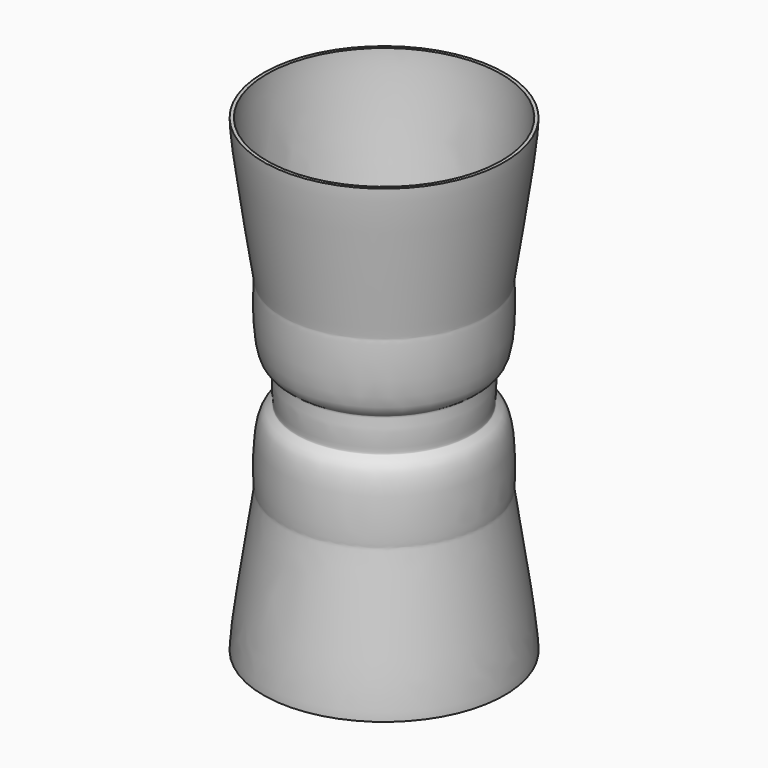
from build123d import *


# Not quite as in the source:
# - the dataset's text gives a spline's control points without its knots; the knots are read off the source's solid


with BuildPart() as f1:
    # F0 (on Front) → F1 (revolve)
    with BuildSketch(Plane.XZ):
        with BuildLine():
            add(Edge.make_bspline(
                [(-25.6999999929, 49.9995985946), (-25.6999852443, 49.5815721843), (-25.6538749277, 48.5653157161), (-25.4124525948, 45.8668468324), (-24.878392708, 41.4753136074), (-24.1648894445, 36.3890603498), (-23.5646349571, 32.3122072602), (-23.1193375058, 29.352931232), (-22.6985490396, 26.594557592), (-22.3219193496, 24.139852673), (-22.0091222222, 22.0915768733), (-21.8182230906, 20.8108258495), (-21.7174489533, 20.0942392935), (-21.67125295, 19.7339820401), (-21.6557990976, 19.5482726937), (-21.6565288364, 19.4907810276), (-21.6608822965, 19.4278153928), (-21.6708680053, 19.3301556268), (-21.6927063082, 19.1336817496), (-21.7207099556, 18.7606404993), (-21.7568005161, 18.0992294459), (-21.7964158924, 16.9880468241), (-21.8179345694, 15.3198351183), (-21.796108146, 13.4398535012), (-21.7132440964, 11.4715337789), (-21.5509831384, 9.5365922757), (-21.3331419094, 8.0502720792), (-21.0956507165, 6.9899388657), (-20.9159406074, 6.3893416768), (-20.7487018006, 5.9506466857), (-20.5613811169, 5.5380982544), (-20.2931757466, 5.0927515424), (-19.9384796595, 4.6682731625), (-19.5759422383, 4.3410734286), (-19.2352502373, 4.0939290526), (-18.9441027544, 3.9056385832), (-18.727928559, 3.7593647128), (-18.6286459873, 3.6717813487), (-18.5923884128, 3.6276224499), (-18.5741459494, 3.5991000841), (-18.5413846399, 3.5234207305), (-18.5092785415, 3.3386711833), (-18.5010370978, 3.0632052381), (-18.5186377506, 2.7098792723), (-18.5683738347, 2.1473494462), (-18.657056361, 1.2888816597), (-18.7, 0.453140888), (-18.7, 0)],
                knots=[1e-05, 1e-05, 1e-05, 1e-05, 0.03125, 0.0625, 0.125, 0.1875, 0.21875, 0.25, 0.28125, 0.3125, 0.34375, 0.375, 0.390625, 0.40625, 0.421875, 0.4375, 0.4453125, 0.453125, 0.46875, 0.484375, 0.5, 0.53125, 0.5625, 0.59375, 0.625, 0.65625, 0.6875, 0.703125, 0.71875, 0.7265625, 0.734375, 0.75, 0.765625, 0.78125, 0.796875, 0.8125, 0.828125, 0.84375, 0.8515625, 0.859375, 0.875, 0.890625, 0.90625, 0.921875, 0.9375, 0.96875, 1, 1, 1, 1], degree=3))
            Line((-18.7, 0), (-18, 0))
            add(Edge.make_bspline(
                [(-25, 50), (-25, 45), (-20.7458853577, 19.1793841739), (-21.079257979, 19.6349945691), (-21.4844424281, 4.9074373991), (-17.1919062111, 4.4391883758), (-18, 2), (-18, 0)],
                knots=[0, 0, 0, 0, 0.3988240253, 0.4713189234, 0.7330888037, 0.8550102037, 1, 1, 1, 1], degree=3))
            Line((-25, 50), (-25.6999999928, 49.9995985946))
        make_face()
        with BuildLine():
            Line((-25.7, -50), (-25, -50))
            add(Edge.make_bspline(
                [(-25, -50), (-25, -45), (-20.7458853577, -19.1793841739), (-21.079257979, -19.6349945691), (-21.3761518713, -8.8435592571), (-20, -6)],
                knots=[0, 0, 0, 0, 0.3988240253, 0.4713189234, 0.7330888037, 0.7330888037, 0.7330888037, 0.7330888037], degree=3))
            add(Edge.make_bspline(
                [(-20, -6), (-19.5032922638, -4.9736467966), (-18.7970130134, -4.6778168777), (-18.3324850568, -4.3324850568)],
                knots=[0.7330888037, 0.7330888037, 0.7330888037, 0.7330888037, 0.8275719254, 0.8275719254, 0.8275719254, 0.8275719254], degree=3))
            Line((-18.3324850568, -4.3324850568), (-18, -4))
            add(Edge.make_bspline(
                [(-18, -4), (-17.5610324502, -3.3250003398), (-18, -2), (-18, 0)],
                knots=[0.8550102037, 0.8550102037, 0.8550102037, 0.8550102037, 1, 1, 1, 1], degree=3))
            Line((-18, 0), (-18.7, 0))
            add(Edge.make_bspline(
                [(-25.7, -50), (-25.7, -49.5818974293), (-25.653894243, -48.5655316105), (-25.4124525948, -45.8668468324), (-24.878392708, -41.4753136074), (-24.1648894445, -36.3890603498), (-23.5646349571, -32.3122072602), (-23.1193375058, -29.352931232), (-22.6985490396, -26.594557592), (-22.3219193496, -24.139852673), (-22.0091222222, -22.0915768733), (-21.8182230906, -20.8108258495), (-21.7174489533, -20.0942392935), (-21.67125295, -19.7339820401), (-21.6557990976, -19.5482726937), (-21.6565288364, -19.4907810276), (-21.6608822965, -19.4278153928), (-21.6708680053, -19.3301556268), (-21.6927063082, -19.1336817496), (-21.7207099556, -18.7606404993), (-21.7568005161, -18.0992294459), (-21.7964158924, -16.9880468241), (-21.8179345694, -15.3198351183), (-21.796108146, -13.4398535012), (-21.7132440964, -11.4715337789), (-21.5509831384, -9.5365922757), (-21.3331419094, -8.0502720792), (-21.0956507165, -6.9899388657), (-20.9159406074, -6.3893416768), (-20.7487018006, -5.9506466857), (-20.5613811169, -5.5380982544), (-20.2931757466, -5.0927515424), (-19.9384796595, -4.6682731625), (-19.5759422383, -4.3410734286), (-19.2352502373, -4.0939290526), (-18.9441027544, -3.9056385832), (-18.727928559, -3.7593647128), (-18.6286459873, -3.6717813487), (-18.5923884128, -3.6276224499), (-18.5741459494, -3.5991000841), (-18.5413846399, -3.5234207305), (-18.5092785415, -3.3386711833), (-18.5010370978, -3.0632052381), (-18.5186377506, -2.7098792723), (-18.5683738347, -2.1473494462), (-18.657056361, -1.2888816597), (-18.7, -0.453140888), (-18.7, 0)],
                knots=[0, 0, 0, 0, 0.03125, 0.0625, 0.125, 0.1875, 0.21875, 0.25, 0.28125, 0.3125, 0.34375, 0.375, 0.390625, 0.40625, 0.421875, 0.4375, 0.4453125, 0.453125, 0.46875, 0.484375, 0.5, 0.53125, 0.5625, 0.59375, 0.625, 0.65625, 0.6875, 0.703125, 0.71875, 0.7265625, 0.734375, 0.75, 0.765625, 0.78125, 0.796875, 0.8125, 0.828125, 0.84375, 0.8515625, 0.859375, 0.875, 0.890625, 0.90625, 0.921875, 0.9375, 0.96875, 1, 1, 1, 1], degree=3))
        make_face()
    revolve(axis=Axis((0, 0, -25), (0, 0, 1)))


solid = f1.part
